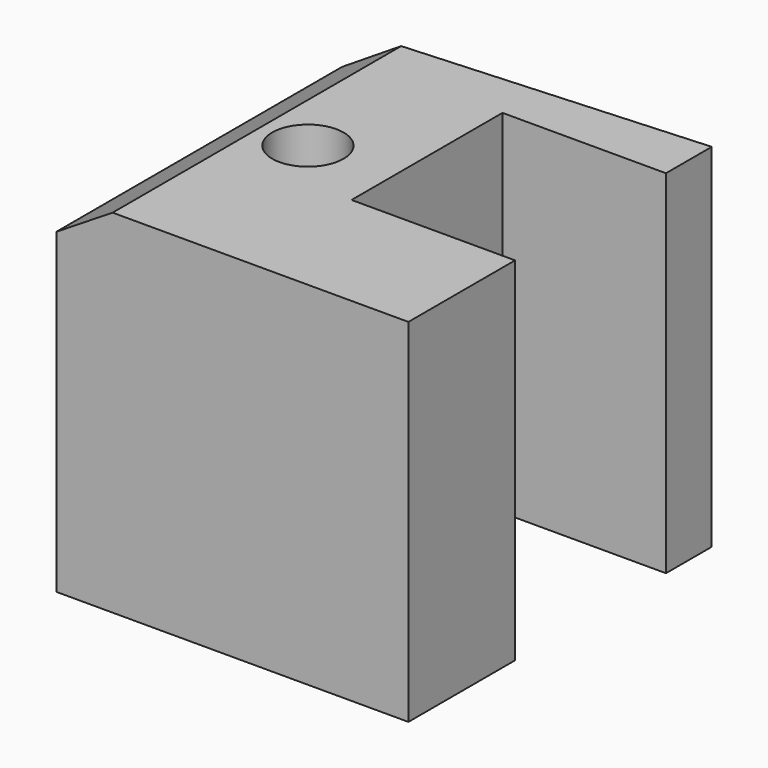
from build123d import *

# Parameters (mm, degrees)
F0_R        = 5.0651423349
F1_DEPTH    = 50
F2_SIZE2    = 8
F2_SIZE     = 5
F4_T1_DEPTH = 460.97003859


# Not quite as in the source:
# - a fillet or chamfer that OpenCascade refuses, or shapes differently, is made with other operations: its cross-section is extruded or revolved along the edge and cut away or added


with BuildPart() as f1:
    # F0 (on Top) → F1 (new body)
    with BuildSketch(Plane.XY):
        Polygon((-70.2088537009, 12.9954309589), (-70.2088537009, 39.781139965), (-46.9945719463, 39.781139965), (-46.9945719463, 49.781139965), (-96.9945719463, 49.781139965), (-96.9945719463, -5.9331371699), (-46.9945719463, -5.9331371699), (-46.9945719463, 12.9954309589), align=None)
        with Locations((-82.137003541, 20.1600026339)):
            Circle(F0_R, mode=Mode.SUBTRACT)
    extrude(amount=F1_DEPTH)

    # F2
    f2_edges = [f1.edges().sort_by_distance(p)[0] for p in [
        (-96.994572, 21.924001, 50),
    ]]
    f2_side = f1.faces().sort_by_distance((-96.994572, 21.924001, 25))[0]
    chamfer(f2_edges, length=F2_SIZE, length2=F2_SIZE2, reference=f2_side)

    # F3: fillet of radius 15 on 1 edges, made by hand

    # F3_s1 → F3_t2 (revolve, cut)
    with BuildSketch(Plane.XZ.offset(-20.1600026339)):
        with BuildLine():
            ThreePointArc((-62.0718612061, 0), (-72.6784629239, 4.3933982822), (-77.0718612061, 15))
            Line((-77.0718612061, 15), (-77.0718612061, 0))
            Line((-77.0718612061, 0), (-62.0718612061, 0))
        make_face()
    revolve(axis=Axis((-82.137003541, 20.1600026339, 0), (0, 0, 1)), mode=Mode.SUBTRACT)

    # F4: chamfer of 5 x 80 on 1 edges, made by hand

    # F4_s2 → F4_t1 (cut)
    with BuildSketch(Plane.XY.offset(-207.985019295)):
        Polygon((-16.9945719463, 49.781139965), (-96.9945719463, 44.781139965), (-96.9945719463, 49.781139965), align=None)
    extrude(amount=F4_T1_DEPTH, mode=Mode.SUBTRACT)


solid = f1.part
